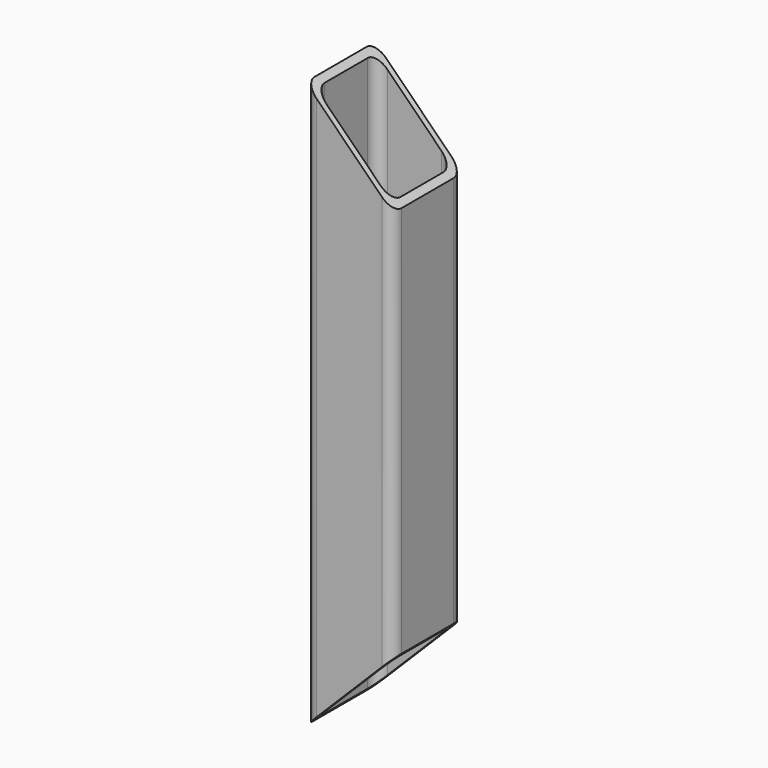
from build123d import *

# Parameters (mm, degrees)
F1_W     = 25.4
F1_H     = 25.4
F2_DEPTH = 165.1
F4_DEPTH = 25.4
F5_R     = 3.175


# Not quite as in the source:
# - a variable given as a bare number and used for a length is read in inches; the dataset says mm whatever the document's units were


with BuildPart() as f2:
    # F1 (on Top) → F2 (new body)
    with BuildSketch(Plane.XY):
        Rectangle(F1_W, F1_H)
        with BuildLine():
            ThreePointArc((-11.049, 7.874), (-10.1190640303, 10.1190640303), (-7.874, 11.049))
            Line((-7.874, 11.049), (7.874, 11.049))
            ThreePointArc((7.874, 11.049), (10.1190640303, 10.1190640303), (11.049, 7.874))
            Line((11.049, 7.874), (11.049, -7.874))
            ThreePointArc((11.049, -7.874), (10.1190640303, -10.1190640303), (7.874, -11.049))
            Line((7.874, -11.049), (-7.874, -11.049))
            ThreePointArc((-7.874, -11.049), (-10.1190640303, -10.1190640303), (-11.049, -7.874))
            Line((-11.049, -7.874), (-11.049, 7.874))
        make_face(mode=Mode.SUBTRACT)
    extrude(amount=F2_DEPTH)

    # F3 (on face) → F4 (cut)
    with BuildSketch(Plane.XZ.offset(12.7)):
        Polygon((12.7, 25.4), (-12.7, 0), (12.7, 0), align=None)
        Polygon((12.7, 165.1), (-12.7, 165.1), (12.7, 139.7), align=None)
    extrude(amount=-F4_DEPTH, mode=Mode.SUBTRACT)

    # F5
    f5_edges = [f2.edges().sort_by_distance(p)[0] for p in [
        (-12.7, 12.7, 82.55),
        (12.7, 12.7, 82.55),
        (-12.7, -12.7, 82.55),
        (12.7, -12.7, 82.55),
    ]]
    fillet(f5_edges, radius=F5_R)


solid = f2.part
